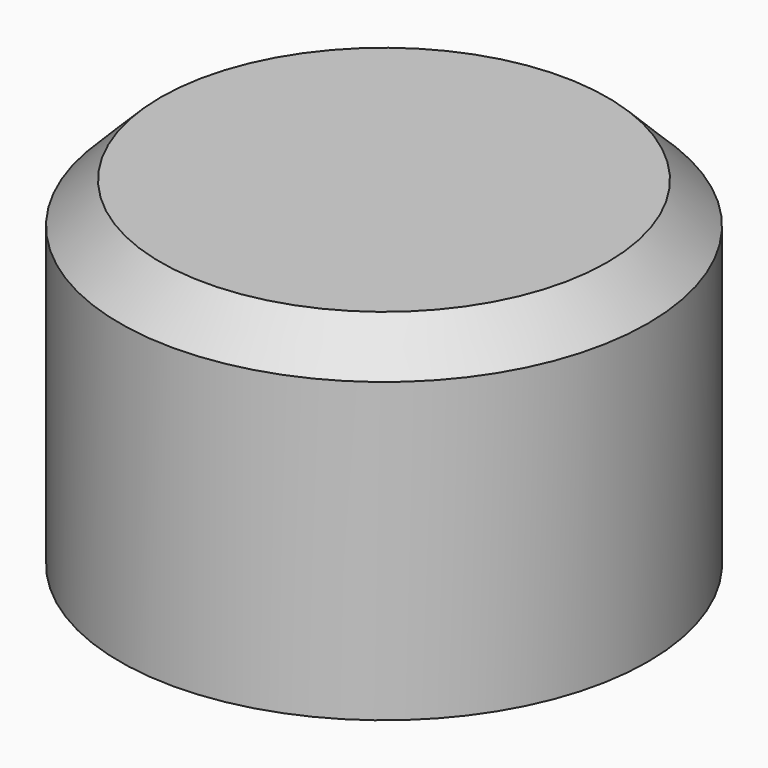
from build123d import *

# Parameters (mm, degrees)
F3_W       = 0.75
F3_H       = 1.9961989338
F5_SIZE2   = 8.144336
F5_SIZE    = 0.99999
F5_2_SIZE2 = 8.144336
F5_2_SIZE  = 0.99999
F5_3_SIZE2 = 8.144336
F5_3_SIZE  = 0.99999


# Not quite as in the source:
# - a fillet or chamfer is up to 0.001 mm smaller than in the source, because OpenCascade refuses the exact size


with BuildPart() as f1:
    # F0 (on Front) → F1 (revolve)
    with BuildSketch(Plane.XZ):
        Polygon((16.5, 25), (0, 25), (0, 23), (12.8431457505, 23), (17.5, 18.3431457505), (17.5, 1), (18.5, 0), (19.5, 0), (19.5, 22), align=None)
    revolve(axis=Axis((0, 0, 16.9686058983), (0, 0, 1)))

    # F3 (on offset) → F4 (join, up to the next surface of F1)
    with BuildSketch(Plane.XY.offset(2)):
        with Locations((0, -17.4980994669)):
            Rectangle(F3_W, F3_H)
        Polygon((16.2056781502, 8.9233399405), (15.8306781502, 9.5728589933), (14.1019191624, 8.5747595264), (14.4769191624, 7.9252404736), align=None)
        Polygon((-15.8306781502, 9.5728589933), (-16.2056781502, 8.9233399405), (-14.4769191624, 7.9252404736), (-14.1019191624, 8.5747595264), align=None)
    extrude(until=Until.NEXT)

    # F5 (size 1 and 8.144346428 in the source; OpenCascade refuses exactly that, so slightly less here)
    f5_edges = [f1.edges().sort_by_distance(p)[0] for p in [
        (0, -16.5, 2),
    ]]
    f5_side = f1.faces().sort_by_distance((0, -16.999331, 2))[0]
    chamfer(f5_edges, length=F5_SIZE, length2=F5_SIZE2, reference=f5_side)

    # F5#2 (size 1 and 8.144346428 in the source; OpenCascade refuses exactly that, so slightly less here)
    f5_2_edges = [f1.edges().sort_by_distance(p)[0] for p in [
        (14.289419, 8.25, 2),
    ]]
    f5_2_side = f1.faces().sort_by_distance((14.721853, 8.499666, 2))[0]
    chamfer(f5_2_edges, length=F5_2_SIZE, length2=F5_2_SIZE2, reference=f5_2_side)

    # F5#3 (size 1 and 8.144346428 in the source; OpenCascade refuses exactly that, so slightly less here)
    f5_3_edges = [f1.edges().sort_by_distance(p)[0] for p in [
        (-14.289419, 8.25, 2),
    ]]
    f5_3_side = f1.faces().sort_by_distance((-14.721853, 8.499666, 2))[0]
    chamfer(f5_3_edges, length=F5_3_SIZE, length2=F5_3_SIZE2, reference=f5_3_side)


solid = f1.part
